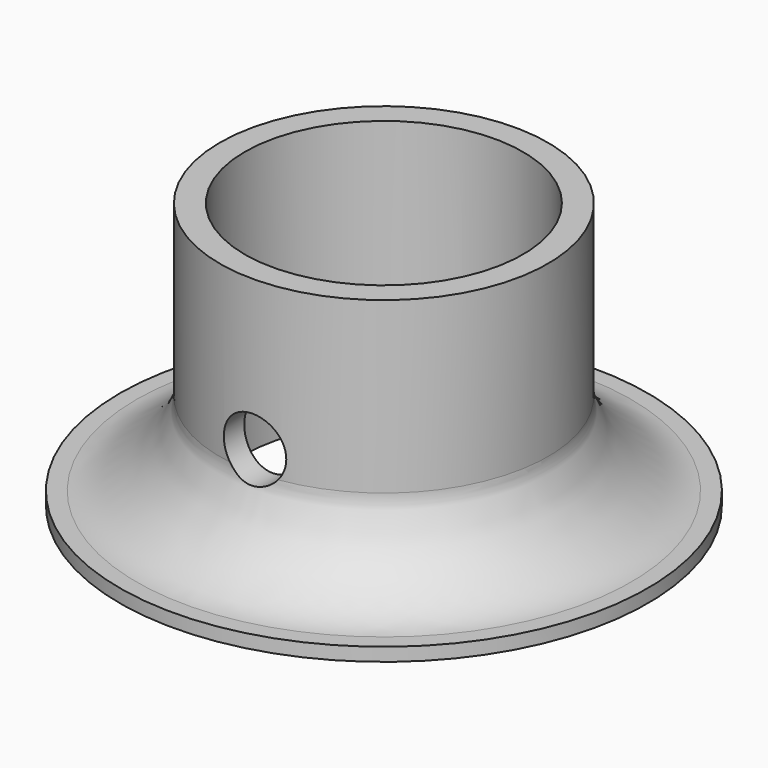
from build123d import *

# Parameters (mm, degrees)
F0_R          = 1.875
F3_DEPTH      = 15.851
F3_DEPTH_BACK = 15.851


# Not quite as in the source:
# - a fillet or chamfer that OpenCascade refuses, or shapes differently, is made with other operations: its cross-section is extruded or revolved along the edge and cut away or added


with BuildPart() as f1:
    # F0 (on Front) → F1 (revolve)
    with BuildSketch(Plane.XZ):
        Polygon((-15.85, 0.8), (-15.85, 0), (-14.35, 0), (-14.35, 0.2), (-11.35, 0.2), (-11.35, 0), (-8.35, 0), (-8.35, 16), (-9.85, 16), (-9.85, 0.8), align=None)
    revolve(axis=Axis((0, 0, 8), (0, 0, 1)))

    # F2: fillet of radius 5 on 1 edges, made by hand

    # F2_s1 → F2_t2 (revolve)
    with BuildSketch(Plane.XZ):
        with BuildLine():
            add(Edge.make_bspline(
                [(-14.85, 0.8), (-9.85, 0.8), (-9.85, 5.8)],
                knots=[0, 0, 0, 1, 1, 1], degree=2, weights=[1, 0.4285714286, 1]))
            Line((-9.85, 5.8), (-9.85, 0.8))
            Line((-9.85, 0.8), (-14.85, 0.8))
        make_face()
    revolve(axis=Axis((0, 0, 0.8), (0, 0, 1)))

    # F0 (on Front) → F3 (cut, two sides)
    with BuildSketch(Plane.XZ) as f3_sk:
        with Locations((0, 7)):
            Circle(F0_R)
    extrude(amount=-F3_DEPTH, mode=Mode.SUBTRACT)
    extrude(f3_sk.sketch, amount=F3_DEPTH_BACK, mode=Mode.SUBTRACT)


solid = f1.part
